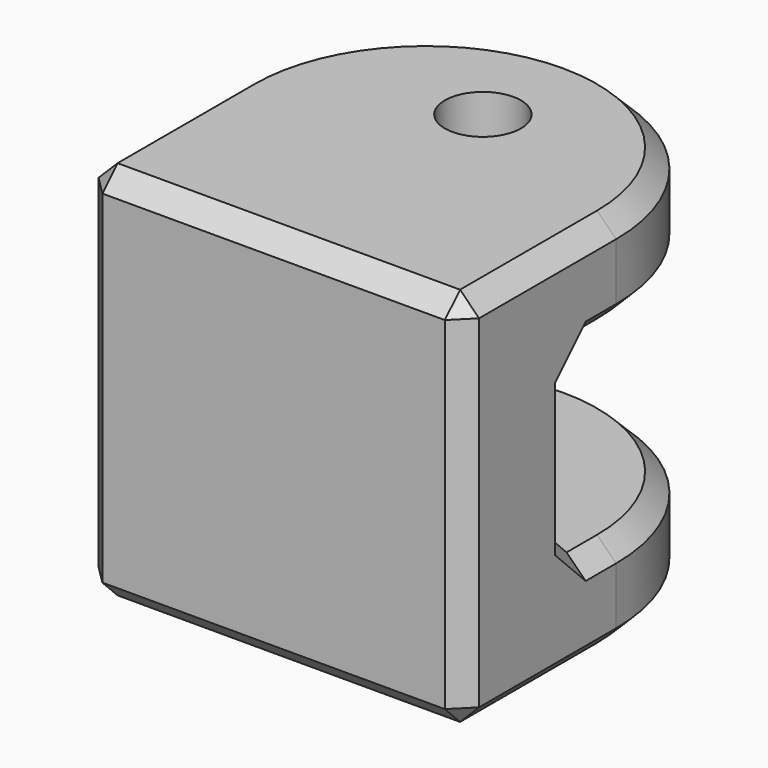
from build123d import *

# Parameters (mm, degrees)
F0_W     = 20
F0_H     = 20
F1_DEPTH = 20
F2_W     = 13
F2_H     = 10
F3_DEPTH = 20
F4_R     = 2
F5_DEPTH = 20
F6_R     = 9.99999
F7_SIZE  = 1


# Not quite as in the source:
# - a fillet or chamfer is up to 0.001 mm smaller than in the source, because OpenCascade refuses the exact size


with BuildPart() as f1:
    # F0 (on Front) → F1 (new body)
    with BuildSketch(Plane.XZ):
        with Locations((10, 10)):
            Rectangle(F0_W, F0_H)
    extrude(amount=-F1_DEPTH)

    # F2 (on face) → F3 (cut, through all)
    with BuildSketch(Plane.YZ.offset(20)):
        with Locations((13.5, 10)):
            Rectangle(F2_W, F2_H)
    extrude(amount=-F3_DEPTH, mode=Mode.SUBTRACT)

    # F4 (on face) → F5 (cut, through all)
    with BuildSketch(Plane.XY.offset(20)):
        with Locations((10, 13.75)):
            Circle(F4_R)
    extrude(amount=-F5_DEPTH, mode=Mode.SUBTRACT)

    # F6 (radius 10 in the source; OpenCascade refuses exactly that, so slightly less here)
    f6_edges = [f1.edges().sort_by_distance(p)[0] for p in [
        (0, 20, 2.5),
        (20, 20, 2.5),
        (20, 20, 17.5),
        (0, 20, 17.5),
    ]]
    fillet(f6_edges, radius=F6_R)

    # F7
    f7_edges = [f1.edges().sort_by_distance(p)[0] for p in [
        (0, 0, 10),
        (10, 0, 0),
        (20, 0, 10),
        (10, 0, 20),
        (10, 7, 15),
        (10, 7, 5),
        (20, 7, 10),
        (0, 7, 10),
        (17.071071, 17.071071, 0),
        (10.00001, 20, 2.5),
        (20, 10.00001, 2.5),
        (17.071071, 17.071071, 5),
        (20, 5.000005, 20),
        (20, 10.00001, 17.5),
        (20, 8.500005, 15),
        (20, 5.000005, 0),
        (20, 8.500005, 5),
        (17.071071, 17.071071, 15),
        (10.00001, 20, 17.5),
        (17.071071, 17.071071, 20),
    ]]
    chamfer(f7_edges, length=F7_SIZE)


solid = f1.part
